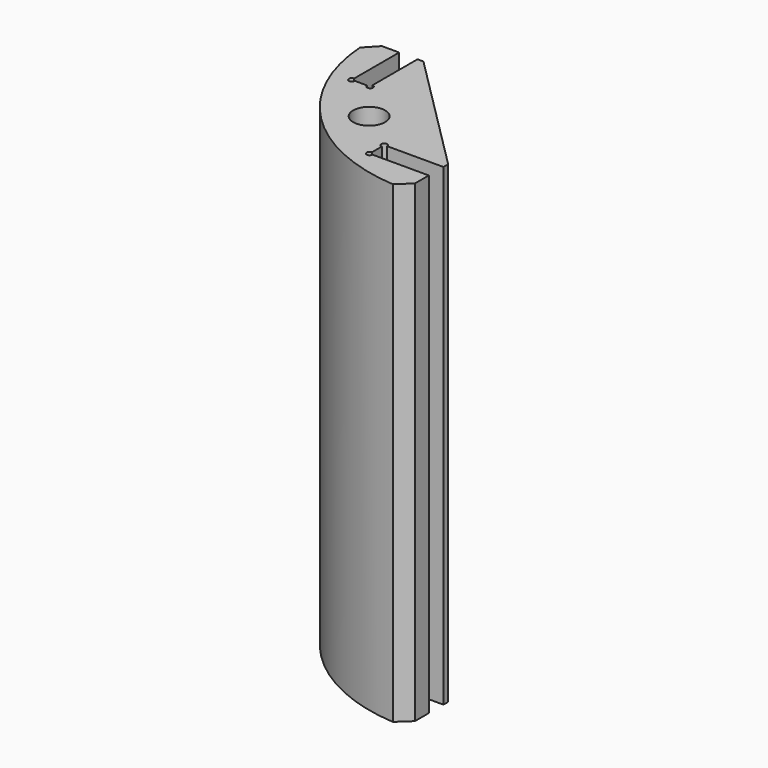
from build123d import *

# Parameters (mm, degrees)
F0_R        = 2.7
F1_DEPTH    = 80
F2_T1_DEPTH = 91.0076112648


# Not quite as in the source:
# - a fillet or chamfer that OpenCascade refuses, or shapes differently, is made with other operations: its cross-section is extruded or revolved along the edge and cut away or added


with BuildPart() as f1:
    # F0 (on Top) → F1 (new body)
    with BuildSketch(Plane.XY):
        with BuildLine():
            Line((-130.9739977717, -74.1217002273), (-135.9739977717, -74.1217002273))
            ThreePointArc((-135.9739977717, -74.1217002273), (-127.1872012073, -95.3349036629), (-105.9739977717, -104.1217002273))
            Line((-105.9739977717, -104.1217002273), (-105.9739977717, -99.1217002273))
            Line((-105.9739977717, -99.1217002273), (-115.4739977717, -99.1217002273))
            ThreePointArc((-115.4739977717, -99.1217002273), (-116.3275511623, -99.4752536179), (-115.9739977717, -98.6217002273))
            Line((-115.9739977717, -98.6217002273), (-115.9739977717, -96.5217002273))
            ThreePointArc((-115.9739977717, -96.5217002273), (-116.3275511623, -95.6681468367), (-115.4739977717, -96.0217002273))
            Line((-115.4739977717, -96.0217002273), (-105.9739977717, -96.0217002273))
            Line((-105.9739977717, -96.0217002273), (-105.9739977717, -95.0217002273))
            Line((-105.9739977717, -95.0217002273), (-126.8739977717, -74.1217002273))
            Line((-126.8739977717, -74.1217002273), (-127.8739977717, -74.1217002273))
            Line((-127.8739977717, -74.1217002273), (-127.8739977717, -83.6217002273))
            ThreePointArc((-127.8739977717, -83.6217002273), (-127.5204443811, -83.7681468367), (-127.3739977717, -84.1217002273))
            ThreePointArc((-127.3739977717, -84.1217002273), (-127.8739977717, -84.6217002273), (-128.3739977717, -84.1217002273))
            Line((-128.3739977717, -84.1217002273), (-130.4739977717, -84.1217002273))
            ThreePointArc((-130.4739977717, -84.1217002273), (-131.3275511623, -84.4752536179), (-130.9739977717, -83.6217002273))
            Line((-130.9739977717, -83.6217002273), (-130.9739977717, -74.1217002273))
        make_face()
        with Locations((-122.684560746, -90.8322632015)):
            Circle(F0_R, mode=Mode.SUBTRACT)
    extrude(amount=F1_DEPTH)

    # F2: chamfer of 2 on 2 edges, made by hand

    # F2_s2 → F2_t1 (cut)
    with BuildSketch(Plane.XY.offset(-5.5038056324)):
        with BuildLine():
            Line((-105.9739977717, -102.0501803148), (-108.1168549146, -104.0450717496))
            ThreePointArc((-108.1168549146, -104.0450717496), (-107.074368306, -104.1015131801), (-105.9739977717, -104.1217002273))
            Line((-105.9739977717, -104.1217002273), (-105.9739977717, -102.0501803148))
        make_face()
        with BuildLine():
            Line((-135.8973692941, -76.2645573701), (-133.9024778593, -74.1217002273))
            Line((-133.9024778593, -74.1217002273), (-135.9739977717, -74.1217002273))
            ThreePointArc((-135.9739977717, -74.1217002273), (-135.9538107246, -75.2220707615), (-135.8973692941, -76.2645573701))
        make_face()
    extrude(amount=F2_T1_DEPTH, mode=Mode.SUBTRACT)


solid = f1.part
